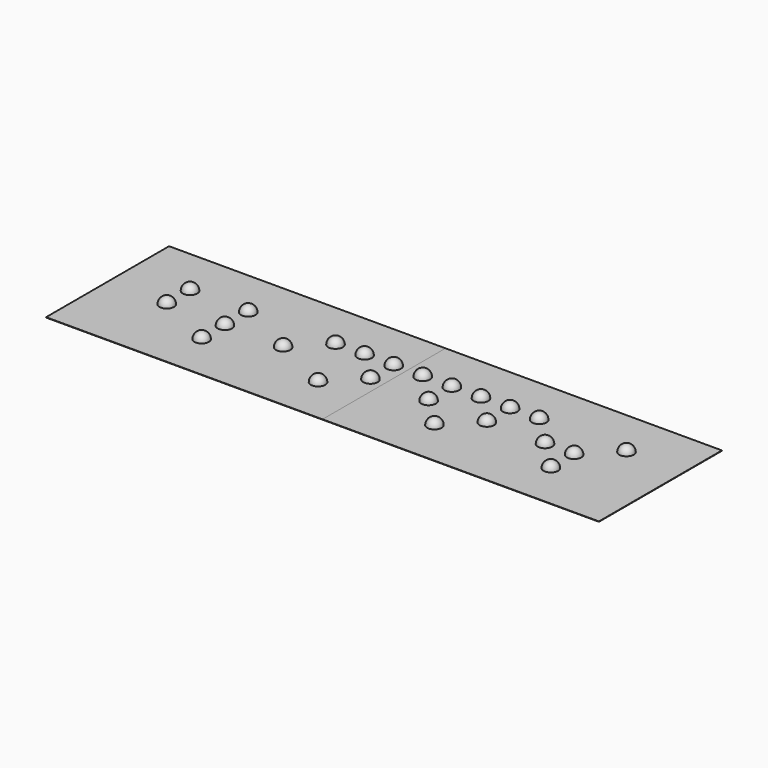
from build123d import *

# Parameters (mm, degrees)
F1_W      = 380
F1_H      = 211.3338357197
F2_DEPTH  = 0.5
F3_R      = 10
F4_DEPTH  = 10
F5_R      = 9.99999
F6_W      = 10
F6_H      = 211.3338357197
F7_DEPTH  = 0.3
F8_W      = 380
F8_H      = 211.3338357197
F9_DEPTH  = 0.5
F10_R     = 10
F11_DEPTH = 10
F12_R     = 9.99999


# Not quite as in the source:
# - a fillet or chamfer is up to 0.001 mm smaller than in the source, because OpenCascade refuses the exact size


with BuildPart() as f2:
    # F1 (on Top) → F2 (new body)
    with BuildSketch(Plane.XY):
        with Locations((-190, 1.3937864294)):
            Rectangle(F1_W, F1_H)
    extrude(amount=F2_DEPTH)

    # F3 (on face) → F4 (join)
    with BuildSketch(Plane.XY.offset(0.5)):
        with Locations((-297.6, 40.0607042892)):
            Circle(F3_R)
        with Locations((-297.6, 0.0607042892)):
            Circle(F3_R)
        with Locations((-217.6, 40.0607042892)):
            Circle(F3_R)
        with Locations((-217.6, 0.0607042892)):
            Circle(F3_R)
        with Locations((-217.6, -39.9392957108)):
            Circle(F3_R)
        with Locations((-137.6, 0.0607042892)):
            Circle(F3_R)
        with Locations((-97.6, 40.0607042892)):
            Circle(F3_R)
        with Locations((-57.6, 40.0607042892)):
            Circle(F3_R)
        with Locations((-57.6, -39.9392957108)):
            Circle(F3_R)
        with Locations((-17.6, 40.0607042892)):
            Circle(F3_R)
        with Locations((-17.6, 0.0607042892)):
            Circle(F3_R)
    extrude(amount=F4_DEPTH)

    # F5 (radius 10 in the source; OpenCascade refuses exactly that, so slightly less here)
    f5_edges = [f2.edges().sort_by_distance(p)[0] for p in [
        (-307.6, 40.060704, 10.5),
        (-307.6, 0.060704, 10.5),
        (-227.6, 40.060704, 10.5),
        (-227.6, 0.060704, 10.5),
        (-227.6, -39.939296, 10.5),
        (-147.6, 0.060704, 10.5),
        (-107.6, 40.060704, 10.5),
        (-67.6, 40.060704, 10.5),
        (-27.6, 40.060704, 10.5),
        (-27.6, 0.060704, 10.5),
        (-67.6, -39.939296, 10.5),
    ]]
    fillet(f5_edges, radius=F5_R)

    # F6 (on face) → F7 (join)
    with BuildSketch(Plane(origin=(0, 0, 0), x_dir=(1, 0, 0), z_dir=(0, 0, -1))):
        with Locations((5, -1.3937864294)):
            Rectangle(F6_W, F6_H)
    extrude(amount=-F7_DEPTH)


with BuildPart() as f9:
    # F8 (on Top) → F9 (new body)
    with BuildSketch(Plane.XY):
        with Locations((190, 1.3937864294)):
            Rectangle(F8_W, F8_H)
    extrude(amount=F9_DEPTH)

    # F10 (on face) → F11 (join)
    with BuildSketch(Plane.XY.offset(0.5)):
        with Locations((22.4, 40.0607042892)):
            Circle(F10_R)
        with Locations((62.4, 40.0607042892)):
            Circle(F10_R)
        with Locations((62.4, 0.0607042892)):
            Circle(F10_R)
        with Locations((102.4, 40.0607042892)):
            Circle(F10_R)
        with Locations((102.4, -39.9392957108)):
            Circle(F10_R)
        with Locations((142.4, 40.0607042892)):
            Circle(F10_R)
        with Locations((142.4, 0.0607042892)):
            Circle(F10_R)
        with Locations((182.4, 40.0607042892)):
            Circle(F10_R)
        with Locations((222.4, 0.0607042892)):
            Circle(F10_R)
        with Locations((262.4, 0.0607042892)):
            Circle(F10_R)
        with Locations((262.4, -39.9392957108)):
            Circle(F10_R)
        with Locations((302.4, 40.0607042892)):
            Circle(F10_R)
    extrude(amount=F11_DEPTH)

    # F12 (radius 10 in the source; OpenCascade refuses exactly that, so slightly less here)
    f12_edges = [f9.edges().sort_by_distance(p)[0] for p in [
        (12.4, 40.060704, 10.5),
        (52.4, 40.060704, 10.5),
        (92.4, 40.060704, 10.5),
        (132.4, 40.060704, 10.5),
        (172.4, 40.060704, 10.5),
        (212.4, 0.060704, 10.5),
        (252.4, 0.060704, 10.5),
        (292.4, 40.060704, 10.5),
        (252.4, -39.939296, 10.5),
        (132.4, 0.060704, 10.5),
        (92.4, -39.939296, 10.5),
        (52.4, 0.060704, 10.5),
    ]]
    fillet(f12_edges, radius=F12_R)


solid = Compound([f2.part, f9.part])
